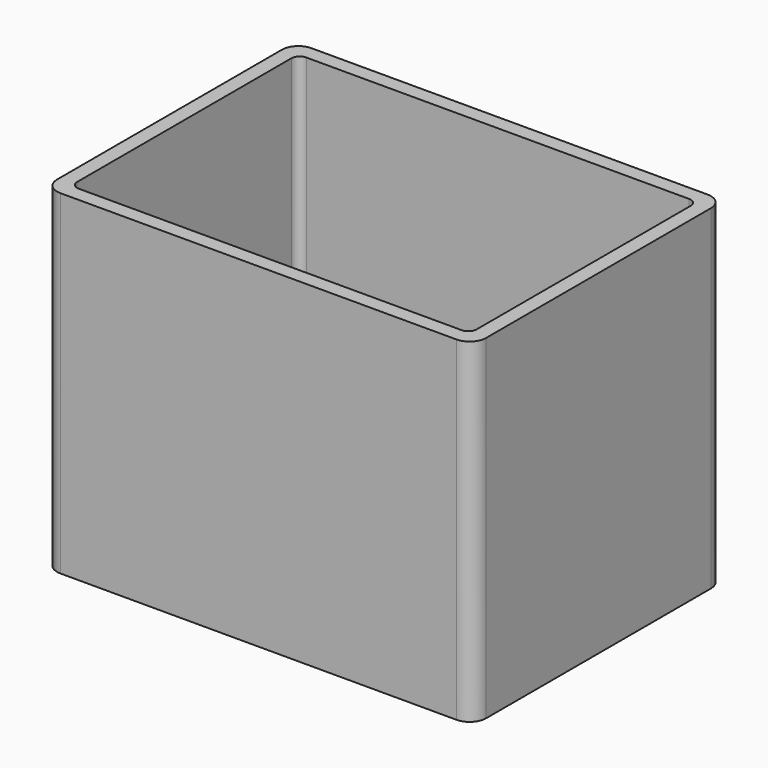
from build123d import *

# Parameters (mm, degrees)
F1_DEPTH = 40.64
F3_DEPTH = 38.608


# Not quite as in the source:
# - a feature names something its author has since deleted; it is built from what else it names


with BuildPart() as f1:
    # F0 (on Top) → F1 (new body)
    with BuildSketch(Plane.XY):
        with BuildLine():
            ThreePointArc((0, 2), (0.5857864376, 0.5857864376), (2, 0))
            Line((2, 0), (50.07, 0))
            ThreePointArc((50.07, 0), (51.4842135624, 0.5857864376), (52.07, 2))
            Line((52.07, 2), (52.07, 36.1))
            ThreePointArc((52.07, 36.1), (51.4842135624, 37.5142135624), (50.07, 38.1))
            Line((50.07, 38.1), (2, 38.1))
            ThreePointArc((2, 38.1), (0.5857864376, 37.5142135624), (0, 36.1))
            Line((0, 36.1), (0, 2))
        make_face()
    extrude(amount=F1_DEPTH)

    # F2 (on face) → F3 (cut)
    with BuildSketch(Plane.XY.offset(40.64)):
        with BuildLine():
            Line((49.27, 36.3), (2.8, 36.3))
            ThreePointArc((2.8, 36.3), (2.0928932188, 36.0071067812), (1.8, 35.3))
            Line((1.8, 35.3), (1.8, 2.8))
            ThreePointArc((1.8, 2.8), (2.0928932188, 2.0928932188), (2.8, 1.8))
            Line((2.8, 1.8), (49.27, 1.8))
            ThreePointArc((49.27, 1.8), (49.9771067812, 2.0928932188), (50.27, 2.8))
            Line((50.27, 2.8), (50.27, 35.3))
            ThreePointArc((50.27, 35.3), (49.9771067812, 36.0071067812), (49.27, 36.3))
        make_face()
    extrude(amount=-F3_DEPTH, mode=Mode.SUBTRACT)


solid = f1.part
